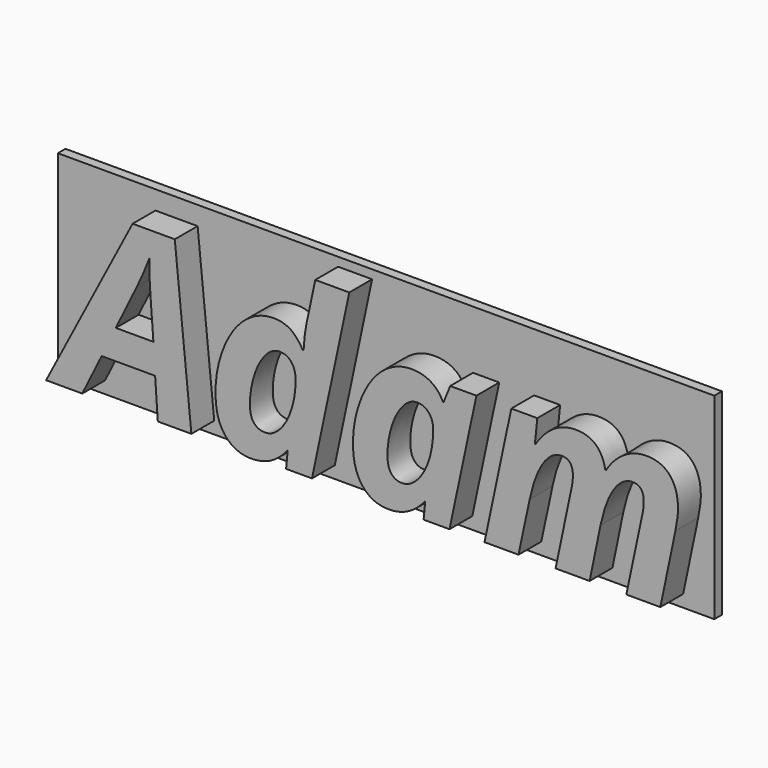
from build123d import *

# Parameters (mm, degrees)
F0_TEXT_SIZE = 24.314187174
F1_DEPTH     = 3
F2_W         = 68.9707361162
F2_H         = 20.673463936
F3_DEPTH     = 1


# Not quite as in the source:
# - Text() gives the source's letters only with a copy of the font that has no kerning and outlines rounded to 1/6400 em; it was checked with that copy


with BuildPart() as f1:
    # F0 (on Front) → F1 (new body)
    with BuildSketch(Plane.XZ):
        with Locations((-44.7518088037, -0.1232831214)):
            Text('Adam', F0_TEXT_SIZE, font='Open Sans', font_style=FontStyle.BOLDITALIC, text_align=(TextAlign.LEFT, TextAlign.BOTTOM))
    extrude(amount=F1_DEPTH)

    # F2 (on face) → F3 (join)
    with BuildSketch(Plane.XZ):
        with Locations((-12.8927920014, 8.9383298182)):
            Rectangle(F2_W, F2_H)
    extrude(amount=-F3_DEPTH)


solid = f1.part
